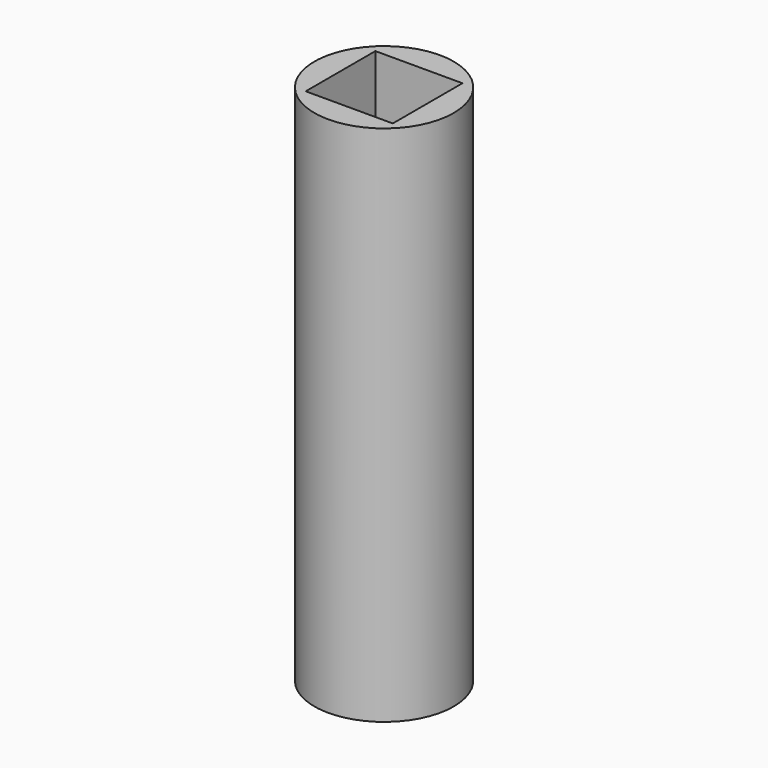
from build123d import *

# Parameters (mm, degrees)
F0_R        = 20
F0_R_2      = 7.5
F1_DEPTH    = 150
F2_W        = 25
F2_H        = 25
F3_DEPTH    = 100
F4_T        = 2.5
F4_T3_DEPTH = 105
F4_T5_DEPTH = 30
F4_T7_DEPTH = 30


# Not quite as in the source:
# - a shell that OpenCascade refuses in one call is made with other operations: the cavity is built on its own and cut out
# - a feature names something its author has since deleted; it is built from what else it names


with BuildPart() as f1:
    # F0 (on Top) → F1 (new body)
    with BuildSketch(Plane.XY):
        Circle(F0_R)
        Circle(F0_R_2, mode=Mode.SUBTRACT)
        Circle(F0_R_2)
    extrude(amount=F1_DEPTH)

    # F2 (on face) → F3 (cut)
    with BuildSketch(Plane.XY.offset(150)):
        Rectangle(F2_W, F2_H)
    extrude(amount=-F3_DEPTH, mode=Mode.SUBTRACT)

    # F4: shell of thickness 2.5, made by hand


with BuildPart() as f4_core1:
    # F4_t2: copy of F1
    add(f1.part)

    # the walls: a layer under each face that stays
    f4_faces = [f4_core1.faces().sort_by_distance(p)[0] for p in [
        (-20, 0, 75),
        (-13.3333333333, -13.3333333333, 150),
        (-12.5, 0, 100),
        (0, -12.5, 100),
        (12.5, 0, 100),
        (0, 12.5, 100),
        (0, 0, 50),
    ]]
    thicken(f4_faces, amount=-F4_T, mode=Mode.SUBTRACT)

    # F4_s4 → F4_t3 (cut)
    with BuildSketch(Plane.XY.offset(47.5)):
        Polygon((-12.475, 12.475), (-15, 12.5), (-15, 15), (-12.5, 15), align=None)
        Polygon((-12.475, -12.475), (-15, -12.5), (-15, -15), (-12.5, -15), align=None)
        Polygon((12.475, -12.475), (12.5, -15), (15, -15), (15, -12.5), align=None)
        Polygon((12.475, 12.475), (15, 12.5), (15, 15), (12.5, 15), align=None)
    extrude(amount=F4_T3_DEPTH, mode=Mode.SUBTRACT)

    # F4_s6 → F4_t5 (cut)
    with BuildSketch(Plane.XZ.offset(-15)):
        Polygon((-12.475, 50.025), (-15, 50), (-15, 47.5), (-12.5, 47.5), align=None)
        Polygon((12.475, 50.025), (15, 50), (15, 47.5), (12.5, 47.5), align=None)
    extrude(amount=F4_T5_DEPTH, mode=Mode.SUBTRACT)

    # F4_s8 → F4_t7 (cut)
    with BuildSketch(Plane.YZ.offset(-15)):
        Polygon((-12.475, 50.025), (-15, 50), (-15, 47.5), (-12.5, 47.5), align=None)
        Polygon((12.475, 50.025), (15, 50), (15, 47.5), (12.5, 47.5), align=None)
    extrude(amount=F4_T7_DEPTH, mode=Mode.SUBTRACT)


with BuildPart() as f1_1:
    add(f1.part)

    # what is left inside the walls is the cavity
    f4_cavity = [f4_core1.part.solids().sort_by_distance(p)[0] for p in [
        (-17.475, 0, 98.333333),
    ]]
    add(f4_cavity, mode=Mode.SUBTRACT)


solid = f1_1.part
